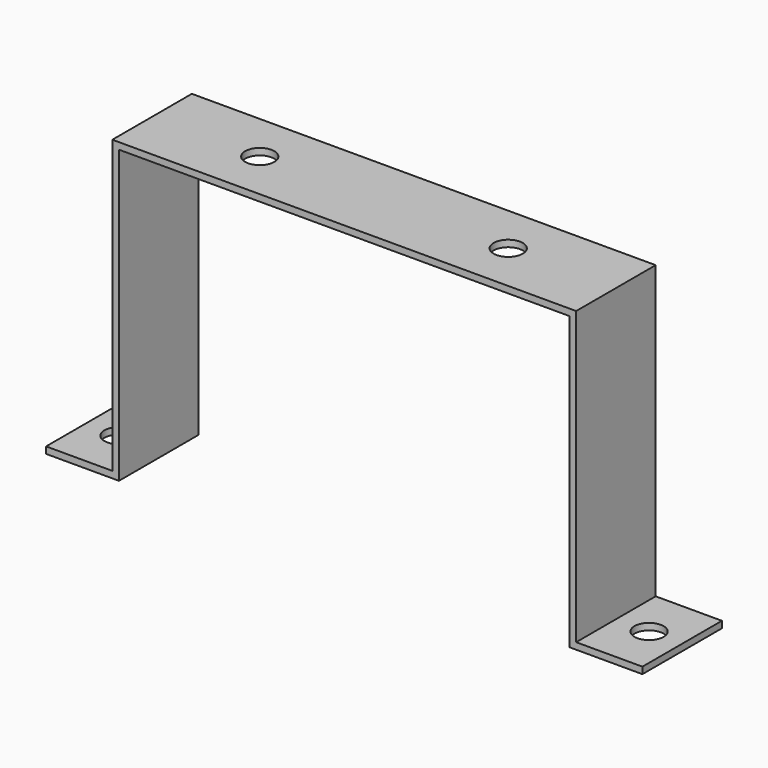
from build123d import *

# Parameters (mm, degrees)
F1_DEPTH = 30
F2_R     = 4.4
F3_R     = 4.4
F4_DEPTH = 25


# Not quite as in the source:
# - a feature names something its author has since deleted; it is built from what else it names


with BuildPart() as f1:
    # F0 (on Front) → F1 (new body)
    with BuildSketch(Plane.XZ):
        Polygon((90, -1), (90, 1), (70, 1), (70, 89), (-70, 89), (-70, 1), (-90, 1), (-90, -1), (-68, -1), (-68, 87), (68, 87), (68, -1), align=None)
    extrude(amount=F1_DEPTH)

    # F2 (on face) + F3 (on face) → F4 (cut)
    with BuildSketch(Plane.XY.offset(1)):
        with Locations((-80, -15)):
            Circle(F2_R)
        with Locations((80, -15)):
            Circle(F2_R)
    with BuildSketch(Plane.XY.offset(89)):
        with Locations((-37.5, -15)):
            Circle(F3_R)
        with Locations((37.5, -15)):
            Circle(F3_R)
    extrude(amount=-F4_DEPTH, mode=Mode.SUBTRACT)


solid = f1.part
